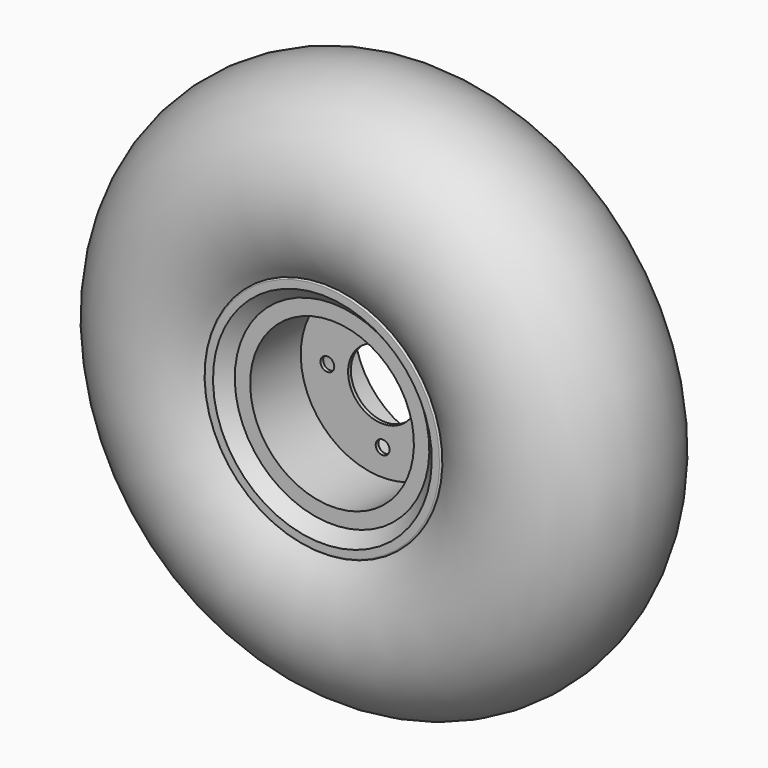
from build123d import *

# Parameters (mm, degrees)
F0_W            = 3.175
F0_H            = 43.4975
F2_R            = 6.35
F3_DEPTH        = 90.4885001
F3_COPIES_COUNT = 4


# Not quite as in the source:
# - a pattern or mirror of a feature is missing from the dataset's text; its kind, count and spacing are read off the source's solid


with BuildPart() as f1:
    # F0 (on Right) → F1 (revolve)
    with BuildSketch(Plane.YZ):
        with BuildLine():
            ThreePointArc((68.2625, 107.6904159243), (68.3373744099, 108.1200376462), (68.5531690141, 108.4990016155))
            ThreePointArc((68.5531690141, 108.4990016155), (0, 254), (-68.5531690141, 108.4990016155))
            ThreePointArc((-68.5531690141, 108.4990016155), (-68.3373744099, 108.1200376462), (-68.2625, 107.6904159243))
            Line((-68.2625, 107.6904159243), (-68.2625, 101.6))
            Line((-68.2625, 101.6), (-57.15, 90.4875))
            Line((-57.15, 90.4875), (-57.15, 77.7875))
            Line((-57.15, 77.7875), (57.15, 77.7875))
            Line((57.15, 77.7875), (57.15, 90.4875))
            Line((57.15, 90.4875), (68.2625, 101.6))
            Line((68.2625, 101.6), (68.2625, 107.6904159243))
        make_face()
        with BuildLine():
            ThreePointArc((70.8025, 107.6904159243), (69.9621217219, 108.8855415143), (68.5531690141, 108.4990016155))
            ThreePointArc((68.5531690141, 108.4990016155), (68.3373744099, 108.1200376462), (68.2625, 107.6904159243))
            Line((68.2625, 107.6904159243), (68.2625, 101.6))
            Line((68.2625, 101.6), (57.15, 90.4875))
            Line((57.15, 90.4875), (57.15, 77.7875))
            Line((57.15, 77.7875), (-57.15, 77.7875))
            Line((-57.15, 77.7875), (-57.15, 90.4875))
            Line((-57.15, 90.4875), (-68.2625, 101.6))
            Line((-68.2625, 101.6), (-68.2625, 107.6904159243))
            ThreePointArc((-68.2625, 107.6904159243), (-68.3373744099, 108.1200376462), (-68.5531690141, 108.4990016155))
            ThreePointArc((-68.5531690141, 108.4990016155), (-69.9621217219, 108.8855415143), (-70.8025, 107.6904159243))
            Line((-70.8025, 107.6904159243), (-70.8025, 100.5478975516))
            Line((-70.8025, 100.5478975516), (-59.69, 89.4353975516))
            Line((-59.69, 89.4353975516), (-59.69, 75.2475))
            Line((-59.69, 75.2475), (-1.5875, 75.2475))
            Line((-1.5875, 75.2475), (1.5875, 75.2475))
            Line((1.5875, 75.2475), (59.69, 75.2475))
            Line((59.69, 75.2475), (59.69, 89.4353975516))
            Line((59.69, 89.4353975516), (70.8025, 100.5478975516))
            Line((70.8025, 100.5478975516), (70.8025, 107.6904159243))
        make_face()
        with Locations((0, 53.49875)):
            Rectangle(F0_W, F0_H)
    revolve(axis=Axis((0, -101.5489548445, 0), (0, -1, 0)))

    # F2 (on face) → F3 (cut, through all)
    with BuildSketch(Plane.XZ.offset(1.5875)):
        with Locations((0, 50.8)):
            Circle(F2_R)
    f3 = extrude(amount=-F3_DEPTH, mode=Mode.SUBTRACT)

    # F3_copies: F3 ×4 about axis
    f3_copies_axis = Axis((0, 0, 0), (0, 1, 0))
    for i in range(1, F3_COPIES_COUNT):
        add(f3.rotate(f3_copies_axis, i * 360 / F3_COPIES_COUNT), mode=Mode.SUBTRACT)


solid = f1.part
